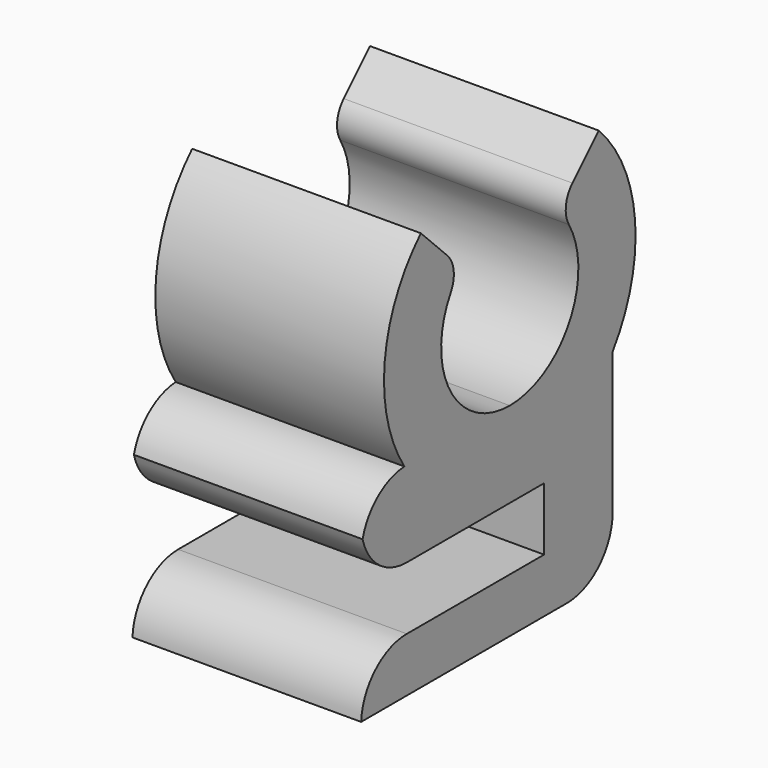
from build123d import *

# Parameters (mm, degrees)
F1_DEPTH    = 4
F2_T1_DEPTH = 10.764079149
F3_W        = 8
F3_H        = 10
F4_DEPTH    = 7
F5_W        = 8
F5_H        = 2.2
F5_W_2      = 11
F5_H_2      = 2.9
F6_DEPTH    = 25
F7_T1_DEPTH = 18
F7_T3_DEPTH = 17.9874921777
F8_W        = 10.9849025458
F8_H        = 7.8663821071
F9_DEPTH    = 25
F11_DEPTH   = 8
F12_R       = 1


# Not quite as in the source:
# - a fillet or chamfer that OpenCascade refuses, or shapes differently, is made with other operations: its cross-section is extruded or revolved along the edge and cut away or added


with BuildPart() as f1:
    # F0 (on Front) → F1 (new body)
    with BuildSketch(Plane.XZ):
        with BuildLine():
            Line((-1.02606043, 2.8190778624), (-1.3680805733, 3.7587704831))
            ThreePointArc((-1.3680805733, 3.7587704831), (-3.2766081772, 2.2943057454), (-4, 0))
            Line((-4, 0), (-4, -8))
            Line((-4, -8), (-4, -13))
            Line((-4, -13), (4, -13))
            Line((4, -13), (4, -3))
            Line((4, -3), (4, 0))
            ThreePointArc((4, 0), (3.2766081772, 2.2943057454), (1.3680805733, 3.7587704831))
            Line((1.3680805733, 3.7587704831), (1.02606043, 2.8190778624))
            ThreePointArc((1.02606043, 2.8190778624), (0, -3), (-1.02606043, 2.8190778624))
        make_face()
    extrude(amount=F1_DEPTH)

    # F2: fillet of radius 1 on 2 edges, made by hand

    # F2_s2 → F2_t1 (cut)
    with BuildSketch(Plane.XZ.offset(-3.3820395745)):
        with BuildLine():
            ThreePointArc((-2.5427622285, 3.087775939), (-1.6437981614, 3.280553188), (-0.9673790506, 2.6578520976))
            Line((-0.9673790506, 2.6578520976), (-1.3680805733, 3.7587704831))
            ThreePointArc((-1.3680805733, 3.7587704831), (-1.9839937688, 3.4732936423), (-2.5427622285, 3.087775939))
        make_face()
        with BuildLine():
            ThreePointArc((2.5427622285, 3.087775939), (1.6437981614, 3.280553188), (0.9673790506, 2.6578520976))
            Line((0.9673790506, 2.6578520976), (1.3680805733, 3.7587704831))
            ThreePointArc((1.3680805733, 3.7587704831), (1.9839937688, 3.4732936423), (2.5427622285, 3.087775939))
        make_face()
    extrude(amount=F2_T1_DEPTH, mode=Mode.SUBTRACT)

    # F3 (on face) → F4 (join)
    with BuildSketch(Plane.XZ.offset(4)):
        with Locations((0, -8)):
            Rectangle(F3_W, F3_H)
    extrude(amount=F4_DEPTH)

    # F5 (on face) → F6 (cut)
    with BuildSketch(Plane.YZ.offset(4)):
        with Locations((-7, -7.1)):
            Rectangle(F5_W, F5_H)
        with Locations((-5.5, -11.55)):
            Rectangle(F5_W_2, F5_H_2)
    extrude(amount=-F6_DEPTH, mode=Mode.SUBTRACT)

    # F7: fillet of radius 2 on 4 edges, made by hand

    # F7_s2 → F7_t1 (cut)
    with BuildSketch(Plane.YZ.offset(-9)):
        with BuildLine():
            ThreePointArc((-11, -4), (-10.4142135624, -5.4142135624), (-9, -6))
            Line((-9, -6), (-11, -6))
            Line((-11, -6), (-11, -4))
        make_face()
        with BuildLine():
            ThreePointArc((-9, -3), (-10.4142135624, -3.5857864376), (-11, -5))
            Line((-11, -5), (-11, -3))
            Line((-11, -3), (-9, -3))
        make_face()
        with BuildLine():
            ThreePointArc((0, -8.1), (-0.5857864376, -9.5142135624), (-2, -10.1))
            Line((-2, -10.1), (0, -10.1))
            Line((0, -10.1), (0, -8.1))
        make_face()
    extrude(amount=F7_T1_DEPTH, mode=Mode.SUBTRACT)

    # F7_s4 → F7_t3 (cut)
    with BuildSketch(Plane.YZ.offset(-8.9937460889)):
        with BuildLine():
            ThreePointArc((-9.0025015645, -8.2), (-10.3809064397, -8.7508623254), (-11, -10.1))
            Line((-11, -10.1), (-11, -8.2))
            Line((-11, -8.2), (-9.0025015645, -8.2))
        make_face()
    extrude(amount=F7_T3_DEPTH, mode=Mode.SUBTRACT)

    # F8 (on face) → F9 (cut)
    with BuildSketch(Plane.XZ.offset(4)):
        with Locations((-1.4924512729, 0.9331910536)):
            Rectangle(F8_W, F8_H)
    extrude(amount=-F9_DEPTH, mode=Mode.SUBTRACT)

    # F10 (on face) → F11 (join, through all)
    with BuildSketch(Plane.YZ.offset(4)):
        with BuildLine():
            ThreePointArc((-2.3786796564, 2.1213203436), (-1.7283614025, -1.1480502971), (-4.5, -3))
            Line((-4.5, -3), (-9.1097722286, -3))
            ThreePointArc((-9.1097722286, -3), (-1.0366594684, -4.2726189114), (-0.6109127035, 3.8890872965))
            Line((-0.6109127035, 3.8890872965), (-2.3786796564, 2.1213203436))
        make_face()
        with BuildLine():
            Line((-9.1097722286, -3), (-4.5, -3))
            ThreePointArc((-4.5, -3), (-7.2716385975, -1.1480502971), (-6.6213203436, 2.1213203436))
            Line((-6.6213203436, 2.1213203436), (-8.3890872965, 3.8890872965))
            ThreePointArc((-8.3890872965, 3.8890872965), (-9.9701493811, 0.5722462303), (-9.1097722286, -3))
        make_face()
    extrude(amount=-F11_DEPTH)

    # F12
    f12_edges = [f1.edges().sort_by_distance(p)[0] for p in [
        (0, -2.37868, 2.12132),
        (0, -6.62132, 2.12132),
    ]]
    fillet(f12_edges, radius=F12_R)


solid = f1.part
